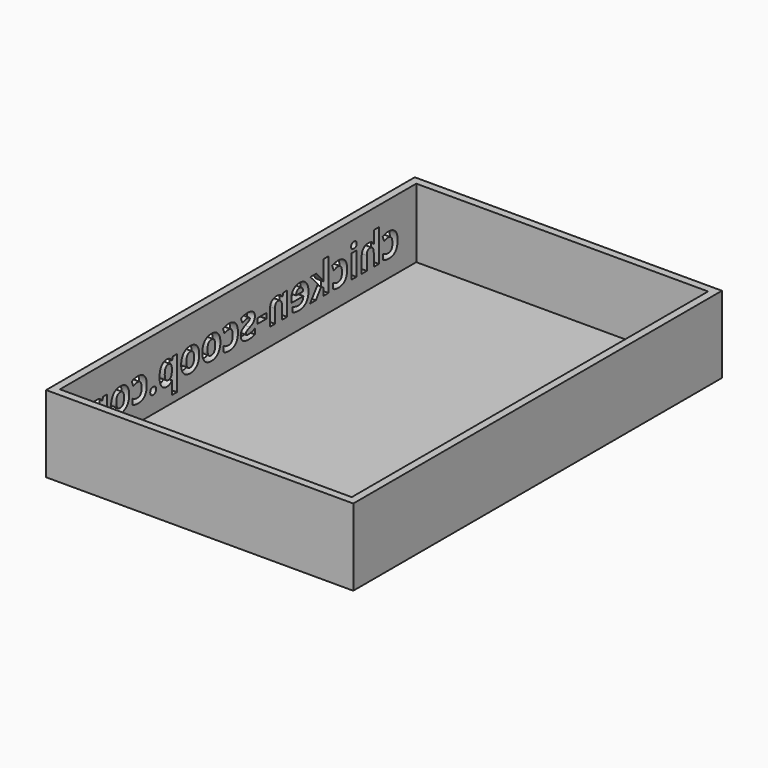
from build123d import *

# Parameters (mm, degrees)
F0_W         = 100
F0_H         = 150
F0_W_2       = 95
F0_H_2       = 145
F1_DEPTH     = 25
F2_DEPTH     = 2.5
F3_TEXT_SIZE = 13.8888888889
F4_DEPTH     = 3


# Not quite as in the source:
# - Text() gives the source's letters only with a copy of the font that has no kerning and outlines rounded to 1/6400 em; it was checked with that copy


with BuildPart() as f1:
    # F0 (on Top) → F1 (new body)
    with BuildSketch(Plane.XY):
        Rectangle(F0_W, F0_H)
        Rectangle(F0_W_2, F0_H_2, mode=Mode.SUBTRACT)
    extrude(amount=F1_DEPTH)

    # F0 (on Top) → F2 (join)
    with BuildSketch(Plane.XY):
        Rectangle(F0_W_2, F0_H_2)
    extrude(amount=F2_DEPTH)

    # F3 (on face) → F4 (cut)
    with BuildSketch(Plane(origin=(-50, 0, 0), x_dir=(0, -1, 0), z_dir=(-1, 0, 0))):
        with Locations((-65.5244124384, 8.1680692358)):
            Text('chicken-scoop.com', F3_TEXT_SIZE, font='Open Sans', font_style=FontStyle.BOLD, text_align=(TextAlign.LEFT, TextAlign.BOTTOM))
    extrude(amount=-F4_DEPTH, mode=Mode.SUBTRACT)


solid = f1.part
